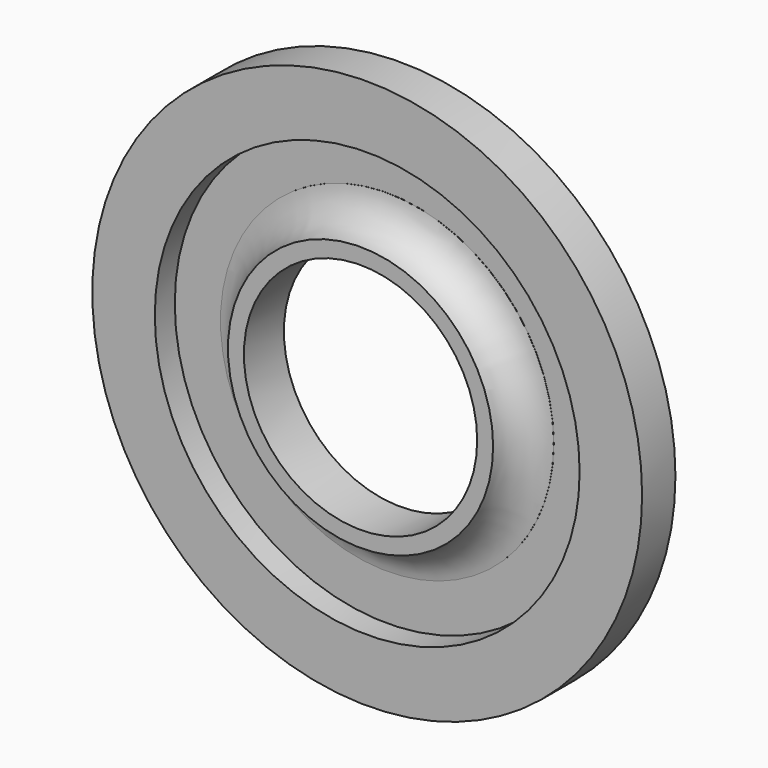
from build123d import *

# Parameters (mm, degrees)
F0_R     = 33
F0_R_2   = 14
F1_DEPTH = 5
F2_R     = 25.5
F2_R_2   = 14
F3_DEPTH = 3
F4_R     = 20
F4_R_2   = 14
F5_DEPTH = 4


with BuildPart() as f1:
    # F0 (on Front) → F1 (new body)
    with BuildSketch(Plane.XZ):
        Circle(F0_R)
        Circle(F0_R_2, mode=Mode.SUBTRACT)
    extrude(amount=F1_DEPTH)

    # F2 (on face) → F3 (cut)
    with BuildSketch(Plane.XZ.offset(5)):
        Circle(F2_R)
        Circle(F2_R_2, mode=Mode.SUBTRACT)
    extrude(amount=-F3_DEPTH, mode=Mode.SUBTRACT)

    # F4 (on face) → F5 (join)
    with BuildSketch(Plane.XZ.offset(2)):
        Circle(F4_R)
        Circle(F4_R_2, mode=Mode.SUBTRACT)
    extrude(amount=F5_DEPTH)

    # F6 (on Top) → F7 (revolve, cut)
    with BuildSketch(Plane.XY):
        with BuildLine():
            ThreePointArc((20.3859657049, -2), (17.2039851896, -9.6819805153), (24.8859657049, -6.5))
            ThreePointArc((24.8859657049, -6.5), (23.5679462203, -3.3180194847), (20.3859657049, -2))
        make_face()
    revolve(axis=Axis((0, -6, 0), (0, -1, 0)), mode=Mode.SUBTRACT)


solid = f1.part
